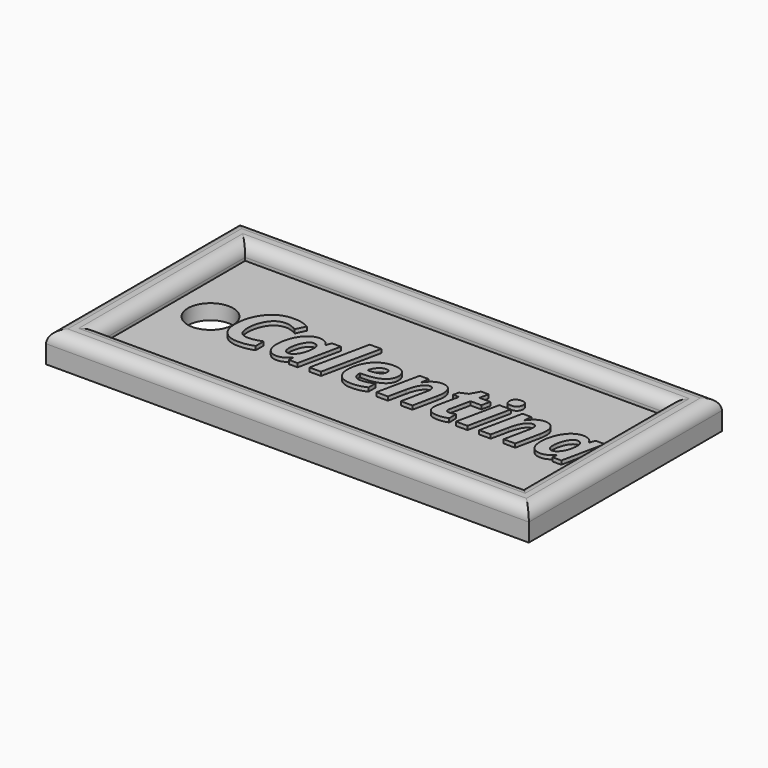
from build123d import *

# Parameters (mm, degrees)
F0_W         = 44.45
F0_H         = 19.05
F0_R         = 2.38125
F1_DEPTH     = 1.5875
F0_W_2       = 50.8
F0_H_2       = 25.4
F2_DEPTH     = 3.175
F3_R         = 1.27
F4_TEXT_SIZE = 8.2514974113
F5_DEPTH     = 0.396875


# Not quite as in the source:
# - Text() gives the source's letters only with a copy of the font that has no kerning and outlines rounded to 1/6400 em; it was checked with that copy


with BuildPart() as f1:
    # F0 (on Top) → F1 (new body)
    with BuildSketch(Plane.XY):
        with Locations((25.4, 12.7)):
            Rectangle(F0_W, F0_H)
        with Locations((7.14375, 12.7)):
            Circle(F0_R, mode=Mode.SUBTRACT)
    extrude(amount=F1_DEPTH)

    # F0 (on Top) → F2 (join)
    with BuildSketch(Plane.XY):
        with Locations((25.4, 12.7)):
            Rectangle(F0_W_2, F0_H_2)
        with Locations((25.4, 12.7)):
            Rectangle(F0_W, F0_H, mode=Mode.SUBTRACT)
    extrude(amount=F2_DEPTH)

    # F3
    f3_edges = [f1.edges().sort_by_distance(p)[0] for p in [
        (25.4, 0, 3.175),
        (0, 12.7, 3.175),
        (25.4, 25.4, 3.175),
        (50.8, 12.7, 3.175),
        (25.4, 22.225, 3.175),
        (3.175, 12.7, 3.175),
        (25.4, 3.175, 3.175),
        (47.625, 12.7, 3.175),
    ]]
    fillet(f3_edges, radius=F3_R)

    # F4 (on face) → F5 (join)
    with BuildSketch(Plane.XY.offset(1.5875)):
        with Locations((9.525, 10.1083652028)):
            Text('Calentina', F4_TEXT_SIZE, font='Open Sans', font_style=FontStyle.BOLDITALIC, text_align=(TextAlign.LEFT, TextAlign.BOTTOM))
    extrude(amount=F5_DEPTH)


solid = f1.part
